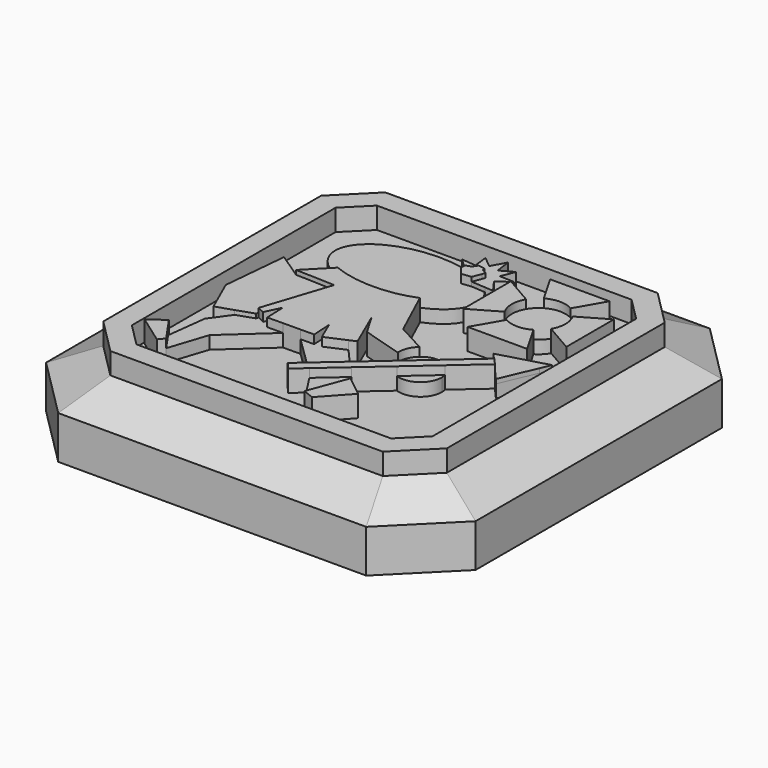
from build123d import *

# Parameters (mm, degrees)
F1_DEPTH    = 3.81
F2_C1_SIZE2 = 2.54
F2_C1_SIZE  = 1.27
F2_C2_SIZE2 = 2.54
F2_C2_SIZE  = 1.27
F2_C3_SIZE2 = 1.27
F2_C3_SIZE  = 2.54
F2_C4_SIZE2 = 1.27
F2_C4_SIZE  = 2.54
F2_C5_SIZE2 = 1.27
F2_C5_SIZE  = 2.54
F2_C6_SIZE2 = 1.27
F2_C6_SIZE  = 2.54
F2_C7_SIZE2 = 1.27
F2_C7_SIZE  = 2.54
F2_C8_SIZE2 = 1.27
F2_C8_SIZE  = 2.54
F4_DEPTH    = 5.08
F6_DEPTH    = 5.08
F7_DEPTH    = 4.572
F9_DEPTH    = 5.08
F10_DEPTH   = 4.826
F11_DEPTH   = 4.572


with BuildPart() as f1:
    # F0 (on Top) → F1 (new body)
    with BuildSketch(Plane.XY):
        Polygon((-12.7, 9.1078975516), (-12.7, 0), (12.7, 0), (12.7, 9.1078975516), (9.1078975516, 12.7), (0, 12.7), (-9.1078975516, 12.7), align=None)
        Polygon((12.7, 0), (-12.7, 0), (-12.7, -9.1078975516), (-9.1078975516, -12.7), (0, -12.7), (9.1078975516, -12.7), (12.7, -9.1078975516), align=None)
    extrude(amount=F1_DEPTH)

    # F2: chamfer of 1.27 x 2.54 on 8 edges, made by hand

    # F2_c1
    f2_c1_edges = [f1.edges().sort_by_distance(p)[0] for p in [
        (10.9039487758, 10.9039487758, 3.81),
    ]]
    f2_c1_side = f1.faces().sort_by_distance((10.9039487758, 10.9039487758, 3.7846))[0]
    chamfer(f2_c1_edges, length=F2_C1_SIZE, length2=F2_C1_SIZE2, reference=f2_c1_side)

    # F2_c2
    f2_c2_edges = [f1.edges().sort_by_distance(p)[0] for p in [
        (-1.7960512242, 12.7, 3.81),
    ]]
    f2_c2_side = f1.faces().sort_by_distance((-1.7960512242, 12.7, 3.7846))[0]
    chamfer(f2_c2_edges, length=F2_C2_SIZE, length2=F2_C2_SIZE2, reference=f2_c2_side)

    # F2_c3
    f2_c3_edges = [f1.edges().sort_by_distance(p)[0] for p in [
        (-12.1739487758, 9.6339487758, 3.81),
    ]]
    f2_c3_side = f1.faces().sort_by_distance((-12.1559882635, 9.6159882635, 3.81))[0]
    chamfer(f2_c3_edges, length=F2_C3_SIZE, length2=F2_C3_SIZE2, reference=f2_c3_side)

    # F2_c4
    f2_c4_edges = [f1.edges().sort_by_distance(p)[0] for p in [
        (-12.7, -1.7960512242, 3.81),
    ]]
    f2_c4_side = f1.faces().sort_by_distance((-12.6746, -1.7960512242, 3.81))[0]
    chamfer(f2_c4_edges, length=F2_C4_SIZE, length2=F2_C4_SIZE2, reference=f2_c4_side)

    # F2_c5
    f2_c5_edges = [f1.edges().sort_by_distance(p)[0] for p in [
        (-9.6339487758, -12.1739487758, 3.81),
    ]]
    f2_c5_side = f1.faces().sort_by_distance((-9.6159882635, -12.1559882635, 3.81))[0]
    chamfer(f2_c5_edges, length=F2_C5_SIZE, length2=F2_C5_SIZE2, reference=f2_c5_side)

    # F2_c6
    f2_c6_edges = [f1.edges().sort_by_distance(p)[0] for p in [
        (1.7960512242, -12.7, 3.81),
    ]]
    f2_c6_side = f1.faces().sort_by_distance((1.7960512242, -12.6746, 3.81))[0]
    chamfer(f2_c6_edges, length=F2_C6_SIZE, length2=F2_C6_SIZE2, reference=f2_c6_side)

    # F2_c7
    f2_c7_edges = [f1.edges().sort_by_distance(p)[0] for p in [
        (12.1739487758, -9.6339487758, 3.81),
    ]]
    f2_c7_side = f1.faces().sort_by_distance((12.1559882635, -9.6159882635, 3.81))[0]
    chamfer(f2_c7_edges, length=F2_C7_SIZE, length2=F2_C7_SIZE2, reference=f2_c7_side)

    # F2_c8
    f2_c8_edges = [f1.edges().sort_by_distance(p)[0] for p in [
        (12.7, 0, 3.81),
    ]]
    f2_c8_side = f1.faces().sort_by_distance((12.6746, 0, 3.81))[0]
    chamfer(f2_c8_edges, length=F2_C8_SIZE, length2=F2_C8_SIZE2, reference=f2_c8_side)

    # F3 (on Top) → F4 (join)
    with BuildSketch(Plane.XY):
        Polygon((-8.0557951031, 10.16), (-10.16, 8.0557951031), (-10.16, 0), (-10.16, -8.0557951031), (-8.0557951031, -10.16), (0, -10.16), (8.0557951031, -10.16), (10.16, -8.0557951031), (10.16, 0), (10.16, 8.0557951031), (8.0557951031, 10.16), (0, 10.16), align=None)
        Polygon((-7.5297438789, 8.89), (0, 8.89), (7.5297438789, 8.89), (8.89, 7.5297438789), (8.89, 0), (8.89, -7.5297438789), (7.5297438789, -8.89), (0, -8.89), (-7.5297438789, -8.89), (-8.89, -7.5297438789), (-8.89, 0), (-8.89, 7.5297438789), align=None, mode=Mode.SUBTRACT)
    extrude(amount=F4_DEPTH)

    # F5 (on Top) → F6 (join)
    with BuildSketch(Plane.XY):
        with BuildLine():
            ThreePointArc((4.28625, 6.4548153285), (5.08, 6.6675), (5.87375, 6.4548153285))
            Line((5.87375, 6.4548153285), (6.8397636205, 8.128))
            Line((6.8397636205, 8.128), (5.08, 8.128))
            Line((5.08, 8.128), (3.3202363795, 8.128))
            Line((3.3202363795, 8.128), (4.28625, 6.4548153285))
        make_face()
        with BuildLine():
            ThreePointArc((3.7051846715, 4.28625), (3.4925, 5.08), (3.7051846715, 5.87375))
            Line((3.7051846715, 5.87375), (2.032, 6.8397636205))
            Line((2.032, 6.8397636205), (2.032, 5.08))
            Line((2.032, 5.08), (2.032, 3.3202363795))
            Line((2.032, 3.3202363795), (3.7051846715, 4.28625))
        make_face()
        with BuildLine():
            Line((6.8397636205, 2.032), (5.87375, 3.7051846715))
            ThreePointArc((5.87375, 3.7051846715), (5.08, 3.4925), (4.28625, 3.7051846715))
            Line((4.28625, 3.7051846715), (3.3202363795, 2.032))
            Line((3.3202363795, 2.032), (5.08, 2.032))
            Line((5.08, 2.032), (6.8397636205, 2.032))
        make_face()
        with BuildLine():
            ThreePointArc((6.4548153285, 5.87375), (6.6134072492, 5.4908752341), (6.6675, 5.08))
            ThreePointArc((6.6675, 5.08), (6.6134072492, 4.6691247659), (6.4548153285, 4.28625))
            Line((6.4548153285, 4.28625), (8.128, 3.3202363795))
            Line((8.128, 3.3202363795), (8.128, 5.08))
            Line((8.128, 5.08), (8.128, 6.8397636205))
            Line((8.128, 6.8397636205), (6.4548153285, 5.87375))
        make_face()
    extrude(amount=F6_DEPTH)

    # F5 (on Top) → F7 (join)
    with BuildSketch(Plane.XY):
        with BuildLine():
            ThreePointArc((6.4548153285, 4.28625), (6.6134072492, 4.6691247659), (6.6675, 5.08))
            ThreePointArc((6.6675, 5.08), (6.6134072492, 5.4908752341), (6.4548153285, 5.87375))
            ThreePointArc((6.4548153285, 5.87375), (6.2025320151, 6.2025320151), (5.87375, 6.4548153285))
            ThreePointArc((5.87375, 6.4548153285), (5.08, 6.6675), (4.28625, 6.4548153285))
            ThreePointArc((4.28625, 6.4548153285), (3.9574679849, 6.2025320151), (3.7051846715, 5.87375))
            ThreePointArc((3.7051846715, 5.87375), (3.4925, 5.08), (3.7051846715, 4.28625))
            ThreePointArc((3.7051846715, 4.28625), (3.9574679849, 3.9574679849), (4.28625, 3.7051846715))
            ThreePointArc((4.28625, 3.7051846715), (5.08, 3.4925), (5.87375, 3.7051846715))
            ThreePointArc((5.87375, 3.7051846715), (6.2025320151, 3.9574679849), (6.4548153285, 4.28625))
        make_face()
    extrude(amount=F7_DEPTH)

    # F8 (on Top) → F9 (join)
    with BuildSketch(Plane.XY):
        with BuildLine():
            Line((-0.1122229733, 7.1412893012), (-0.2283629557, 6.970923168))
            add(Edge.make_bspline(
                [(0.5345230121, 6.5649655092), (0.1954104831, 6.7956865989), (-0.2283629557, 6.970923168)],
                knots=[3.8564349537, 3.8564349537, 3.8564349537, 4.1015137697, 4.1015137697, 4.1015137697], degree=2, weights=[1, 0.9925014369, 1]))
            Line((0.5345230121, 6.5649655092), (0.6090782117, 6.7580132745))
            Line((0.6090782117, 6.7580132745), (0.3096088767, 6.9088116288))
            Line((0.3096088767, 6.9088116288), (0.2684735227, 7.0852804929))
            Line((0.2684735227, 7.0852804929), (-0.1122229733, 7.1412893012))
        make_face()
        with BuildLine():
            add(Edge.make_bspline(
                [(0.5345230121, 6.5649655092), (0.1954104831, 6.7956865989), (-0.2283629557, 6.970923168)],
                knots=[3.8564349537, 3.8564349537, 3.8564349537, 4.1015137697, 4.1015137697, 4.1015137697], degree=2, weights=[1, 0.9925014369, 1]))
            Line((-0.2283629557, 6.970923168), (-0.296480488, 6.8710013293))
            Line((-0.296480488, 6.8710013293), (-0.6060331361, 6.7540844902))
            Line((-0.6060331361, 6.7540844902), (-0.6349986652, 6.4688827842))
            Line((-0.6349986652, 6.4688827842), (-0.2414142946, 5.9886332601))
            Line((-0.2414142946, 5.9886332601), (0.33911434, 6.058988627))
            Line((0.33911434, 6.058988627), (0.5345230121, 6.5649655092))
        make_face()
        with BuildLine():
            add(Edge.make_bspline(
                [(-5.066055874, 2.9146913325), (-2.6377830654, 1.8987875245), (-0.2095102569, 2.9146913325)],
                knots=[0.9544315923, 0.9544315923, 0.9544315923, 2.1871610613, 2.1871610613, 2.1871610613], degree=2, weights=[1, 0.8159852913, 1]))
            Line((-5.066055874, 2.9146913325), (-6.4250563176, 1.5313211978))
            Line((-6.4250563176, 1.5313211978), (-4.1055169559, 1.4521585618))
            Line((-4.1055169559, 1.4521585618), (-5.4060533471, -2.5085740731))
            Line((-5.4060533471, -2.5085740731), (-4.9820523317, -2.7108855791))
            Line((-4.9820523317, -2.7108855791), (-4.5451074799, -1.7951439853))
            Line((-4.5451074799, -1.7951439853), (-4.4973927933, -3.0113308435))
            Line((-4.4973927933, -3.0113308435), (-3.5656666441, -3.0023576035))
            Line((-3.5656666441, -3.0023576035), (-2.5437125486, -2.9925153988))
            Line((-2.5437125486, -2.9925153988), (-1.7411372056, -2.9847859805))
            Line((-1.7411372056, -2.9847859805), (-1.8032029016, -1.8171042278))
            Line((-1.8032029016, -1.8171042278), (-1.3126629405, -2.9480719463))
            Line((-1.3126629405, -2.9480719463), (-0.1458716458, -2.4419940565))
            Line((-0.1458716458, -2.4419940565), (0.2500614016, -2.270264149))
            Line((0.2500614016, -2.270264149), (-0.7346309721, 0))
            Line((-0.7346309721, 0), (0, -1.2611933053))
            Line((0, -1.2611933053), (2.4006810907, -1.9832923998))
            ThreePointArc((2.4006810907, -1.9832923998), (2.4965212882, -1.4006640216), (2.8451042978, -0.9240813362))
            Line((2.8451042978, -0.9240813362), (1.1309832335, 0))
            Line((1.1309832335, 0), (-0.2095102569, 2.9146913325))
        make_face()
        with BuildLine():
            Line((6.267204412, 0.3258485435), (4.6548206917, -1.0884101793))
            ThreePointArc((4.6548206917, -1.0884101793), (4.8131218207, -1.3360068254), (4.9103776631, -1.6133236979))
            Line((4.9103776631, -1.6133236979), (6.6385425071, -0.0975106973))
            Line((6.6385425071, -0.0975106973), (6.267204412, 0.3258485435))
        make_face()
        with BuildLine():
            ThreePointArc((3.230594872, -3.0866996908), (2.9683229648, -2.9541221916), (2.7434756533, -2.7648947276))
            Line((2.7434756533, -2.7648947276), (1.2705439903, -4.0568368542))
            Line((1.2705439903, -4.0568368542), (-0.1650148494, -5.3159984208))
            Line((-0.1650148494, -5.3159984208), (-0.9175296873, -5.9760464355))
            Line((-0.9175296873, -5.9760464355), (-0.5461915922, -6.3994056764))
            Line((-0.5461915922, -6.3994056764), (0.1883373353, -5.755133516))
            Line((0.1883373353, -5.755133516), (1.6489901799, -4.4739614225))
            Line((1.6489901799, -4.4739614225), (3.230594872, -3.0866996908))
        make_face()
        with BuildLine():
            ThreePointArc((4.9103776631, -1.6133236979), (4.8131218207, -1.3360068254), (4.6548206917, -1.0884101793))
            Line((4.6548206917, -1.0884101793), (3.6082134362, -2.0064133952))
            Line((3.6082134362, -2.0064133952), (3.4504520638, -2.2990522365))
            Line((3.4504520638, -2.2990522365), (3.3194892238, -2.2596600205))
            Line((3.3194892238, -2.2596600205), (2.7434756533, -2.7648947276))
            ThreePointArc((2.7434756533, -2.7648947276), (2.9683229648, -2.9541221916), (3.230594872, -3.0866996908))
            Line((3.230594872, -3.0866996908), (4.9103776631, -1.6133236979))
        make_face()
        Polygon((3.4504520638, -2.2990522365), (3.6082134362, -2.0064133952), (3.3194892238, -2.2596600205), align=None)
        Polygon((2.3105391301, -5.3735887632), (2.0478229092, -6.0765111406), (2.3105391301, -7.1321311407), (1.446055714, -7.6865968294), (2.1023775917, -7.9413978383), (3.5530366004, -6.3504930586), align=None)
        Polygon((2.3105391301, -7.1321311407), (2.0478229092, -6.0765111406), (1.446055714, -7.6865968294), align=None)
        Polygon((-7.6812878251, -7.4135377072), (-7.56945104, -6.5005150802), (-7.8814765438, -6.0487459414), (-8.8125388605, -6.6918071059), (-7.1131428704, -7.9040396959), (-6.8300124258, -7.5711184181), align=None)
        Polygon((-6.8300124258, -7.5711184181), (-7.56945104, -6.5005150802), (-7.6812878251, -7.4135377072), align=None)
    extrude(amount=F9_DEPTH)

    # F8 (on Top) → F10 (join)
    with BuildSketch(Plane.XY):
        with BuildLine():
            add(Edge.make_bspline(
                [(-0.2283629557, 6.970923168), (-0.6435529453, 7.1426103543), (-1.1159788346, 7.2510490136)],
                knots=[4.1015137697, 4.1015137697, 4.1015137697, 4.3416766277, 4.3416766277, 4.3416766277], degree=2, weights=[1, 0.9927988845, 1]))
            Line((-1.1159788346, 7.2510490136), (-0.6060331361, 6.7540844902))
            Line((-0.6060331361, 6.7540844902), (-0.296480488, 6.8710013293))
            Line((-0.296480488, 6.8710013293), (-0.2283629557, 6.970923168))
        make_face()
        with BuildLine():
            Line((-1.3980745571, 7.5259637088), (-1.1159788346, 7.2510490136))
            add(Edge.make_bspline(
                [(-0.2283629557, 6.970923168), (-0.6435529453, 7.1426103543), (-1.1159788346, 7.2510490136)],
                knots=[4.1015137697, 4.1015137697, 4.1015137697, 4.3416766277, 4.3416766277, 4.3416766277], degree=2, weights=[1, 0.9927988845, 1]))
            Line((-0.2283629557, 6.970923168), (-0.1122229733, 7.1412893012))
            Line((-0.1122229733, 7.1412893012), (0.2684735227, 7.0852804929))
            Line((0.2684735227, 7.0852804929), (0.3096088767, 6.9088116288))
            Line((0.3096088767, 6.9088116288), (0.6090782117, 6.7580132745))
            Line((0.6090782117, 6.7580132745), (0.5345230121, 6.5649655092))
            add(Edge.make_bspline(
                [(1.1557152111, 6.0042832544), (0.9098218014, 6.3096244697), (0.5345230121, 6.5649655092)],
                knots=[3.5855077583, 3.5855077583, 3.5855077583, 3.8564349537, 3.8564349537, 3.8564349537], degree=2, weights=[1, 0.990838829, 1]))
            Line((1.1557152111, 6.0042832544), (1.6702164355, 5.9698160107))
            Line((1.6702164355, 5.9698160107), (1.1289499234, 6.7206872627))
            Line((1.1289499234, 6.7206872627), (1.8821544945, 7.2636357509))
            Line((1.8821544945, 7.2636357509), (1.0052451398, 7.2994958609))
            Line((1.0052451398, 7.2994958609), (1.3326364569, 8.0945212394))
            Line((1.3326364569, 8.0945212394), (0.575529295, 7.6851258054))
            Line((0.575529295, 7.6851258054), (0.4482462537, 8.6188837886))
            Line((0.4482462537, 8.6188837886), (0, 7.7868243679))
            Line((0, 7.7868243679), (-0.6457308773, 8.3072027192))
            Line((-0.6457308773, 8.3072027192), (-0.5539554404, 7.4453111738))
            Line((-0.5539554404, 7.4453111738), (-1.3980745571, 7.5259637088))
        make_face()
        with BuildLine():
            Line((0.33911434, 6.058988627), (1.1557152111, 6.0042832544))
            add(Edge.make_bspline(
                [(1.1557152111, 6.0042832544), (0.9098218014, 6.3096244697), (0.5345230121, 6.5649655092)],
                knots=[3.5855077583, 3.5855077583, 3.5855077583, 3.8564349537, 3.8564349537, 3.8564349537], degree=2, weights=[1, 0.990838829, 1]))
            Line((0.5345230121, 6.5649655092), (0.33911434, 6.058988627))
        make_face()
        Polygon((-4.1055169559, 1.4521585618), (-6.4250563176, 1.5313211978), (-7.9690862074, 2.570554056), (-8.3284450859, -1.2870644341), (-7.4274151883, -3.3228884812), (-6.4405930293, -2.9883922011), (-5.4537708703, -2.6538959209), (-5.4060533471, -2.5085740731), align=None)
        Polygon((5.6168604642, 1.0672998615), (6.267204412, 0.3258485435), (6.6385425071, -0.0975106973), (7.2888864548, -0.8389620153), (8.1954162974, 1.2680589934), (8.4542247833, 1.8696000475), (7.8240782022, 1.6914182343), align=None)
    extrude(amount=F10_DEPTH)


with BuildPart() as f11:
    # F8 (on Top) → F11 (new body)
    with BuildSketch(Plane.XY):
        Polygon((-4.9820523317, -2.7108855791), (-5.4060533471, -2.5085740731), (-5.4537708703, -2.6538959209), (-6.4405930293, -2.9883922011), (-7.2800260969, -4.1376831941), (-7.56945104, -6.5005150802), (-6.8300124258, -7.5711184181), (-6.0855830088, -5.2922624163), (-3.5656666441, -3.0023576035), (-4.4973927933, -3.0113308435), (-4.5451074799, -1.7951439853), align=None)
    extrude(amount=F11_DEPTH)


with BuildPart() as f11b:
    # F8 (on Top) → F11, piece 2 (new body)
    with BuildSketch(Plane.XY):
        Polygon((-0.1650148494, -5.3159984208), (1.2705439903, -4.0568368542), (-0.1458716458, -2.4419940565), (-1.3126629405, -2.9480719463), (-1.8032029016, -1.8171042278), (-1.7411372056, -2.9847859805), (-2.5437125486, -2.9925153988), align=None)
    extrude(amount=F11_DEPTH)


with BuildPart() as f11c:
    # F8 (on Top) → F11, piece 3 (new body)
    with BuildSketch(Plane.XY):
        Polygon((2.0478229092, -6.0765111406), (1.6489901799, -4.4739614225), (0.1883373353, -5.755133516), (1.446055714, -7.6865968294), align=None)
    extrude(amount=F11_DEPTH)


with BuildPart() as f11d:
    # F8 (on Top) → F11, piece 4 (new body)
    with BuildSketch(Plane.XY):
        with BuildLine():
            Line((3.3194892238, -2.2596600205), (2.4006810907, -1.9832923998))
            ThreePointArc((2.4006810907, -1.9832923998), (2.5045685766, -2.4037019591), (2.7434756533, -2.7648947276))
            Line((2.7434756533, -2.7648947276), (3.3194892238, -2.2596600205))
        make_face()
        with BuildLine():
            ThreePointArc((4.6548206917, -1.0884101793), (3.7844887911, -0.6260154622), (2.8451042978, -0.9240813362))
            Line((2.8451042978, -0.9240813362), (3.8884673268, -1.4865575358))
            Line((3.8884673268, -1.4865575358), (3.6082134362, -2.0064133952))
            Line((3.6082134362, -2.0064133952), (4.6548206917, -1.0884101793))
        make_face()
        with BuildLine():
            Line((3.8884673268, -1.4865575358), (2.8451042978, -0.9240813362))
            ThreePointArc((2.8451042978, -0.9240813362), (2.4965212882, -1.4006640216), (2.4006810907, -1.9832923998))
            Line((2.4006810907, -1.9832923998), (3.3194892238, -2.2596600205))
            Line((3.3194892238, -2.2596600205), (3.6082134362, -2.0064133952))
            Line((3.6082134362, -2.0064133952), (3.8884673268, -1.4865575358))
        make_face()
    extrude(amount=F11_DEPTH)


with BuildPart() as f11e:
    # F8 (on Top) → F11, piece 5 (new body)
    with BuildSketch(Plane.XY):
        with BuildLine():
            ThreePointArc((4.9414609286, -1.8928048862), (4.9336662297, -1.7522026956), (4.9103776631, -1.6133236979))
            Line((4.9103776631, -1.6133236979), (3.230594872, -3.0866996908))
            ThreePointArc((3.230594872, -3.0866996908), (4.3973850146, -2.9359308934), (4.9414609286, -1.8928048862))
        make_face()
    extrude(amount=F11_DEPTH)


with BuildPart() as f11f:
    # F8 (on Top) → F11, piece 6 (new body)
    with BuildSketch(Plane.XY):
        Polygon((5.6168604642, 1.0672998615), (6.267204412, 0.3258485435), (6.6385425071, -0.0975106973), (7.2888864548, -0.8389620153), (8.1954162974, 1.2680589934), (8.4542247833, 1.8696000475), (7.8240782022, 1.6914182343), align=None)
    extrude(amount=F11_DEPTH)


with BuildPart() as f11g:
    # F8 (on Top) → F11, piece 7 (new body)
    with BuildSketch(Plane.XY):
        with BuildLine():
            add(Edge.make_bspline(
                [(-1.1159788346, 7.2510490136), (-6.838419009, 8.5645539558), (-6.838419009, 4.9388865009)],
                knots=[4.3416766277, 4.3416766277, 4.3416766277, 6.2831853072, 6.2831853072, 6.2831853072], degree=2, weights=[1, 0.5646771263, 1]))
            add(Edge.make_bspline(
                [(-6.838419009, 4.9388865009), (-6.838419009, 3.6561856373), (-5.066055874, 2.9146913325)],
                knots=[0, 0, 0, 0.9544315923, 0.9544315923, 0.9544315923], degree=2, weights=[1, 0.8882771706, 1]))
            add(Edge.make_bspline(
                [(-5.066055874, 2.9146913325), (-2.6377830654, 1.8987875245), (-0.2095102569, 2.9146913325)],
                knots=[0.9544315923, 0.9544315923, 0.9544315923, 2.1871610613, 2.1871610613, 2.1871610613], degree=2, weights=[1, 0.8159852913, 1]))
            add(Edge.make_bspline(
                [(-0.2095102569, 2.9146913325), (2.672725209, 4.1205171256), (1.1557152111, 6.0042832544)],
                knots=[2.1871610613, 2.1871610613, 2.1871610613, 3.5855077583, 3.5855077583, 3.5855077583], degree=2, weights=[1, 0.7653744694, 1]))
            Line((1.1557152111, 6.0042832544), (0.33911434, 6.058988627))
            Line((0.33911434, 6.058988627), (-0.2414142946, 5.9886332601))
            Line((-0.2414142946, 5.9886332601), (-0.6349986652, 6.4688827842))
            Line((-0.6349986652, 6.4688827842), (-0.6060331361, 6.7540844902))
            Line((-0.6060331361, 6.7540844902), (-1.1159788346, 7.2510490136))
        make_face()
    extrude(amount=F11_DEPTH)


solid = Compound([f1.part, f11.part, f11b.part, f11c.part, f11d.part, f11e.part, f11f.part, f11g.part])
